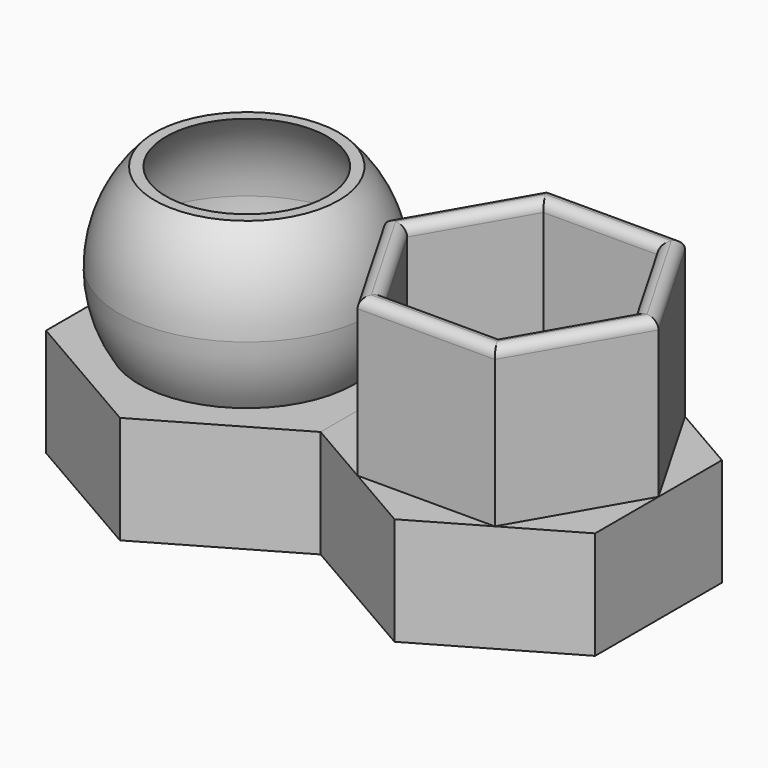
from build123d import *

# Parameters (mm, degrees)
F1_DEPTH        = 34.925
F3_DEPTH        = 50.8
F4_T            = 6.477
F4_T3_DEPTH     = 57.404
F4_T5_DEPTH     = 57.404
F4_T7_DEPTH     = 57.404
F4_T9_DEPTH     = 57.404
F4_T11_DEPTH    = 57.404
F5_R            = 3.23849
F6_R            = 9.5504
F7_DEPTH        = 5.334
F7_COPIES_COUNT = 6
F9_DEPTH        = 34.925
F15_T           = -2.54
F16_W           = 90.7614380121
F16_H           = 120.473433286
F17_DEPTH       = 25.4


# Not quite as in the source:
# - a fillet or chamfer is up to 0.001 mm smaller than in the source, because OpenCascade refuses the exact size
# - a pattern or mirror of a feature is missing from the dataset's text; its kind, count and spacing are read off the source's solid
# - a shell that OpenCascade refuses in one call is made with other operations: the cavity is built on its own and cut out


with BuildPart() as f1:
    # F0 (on Top) → F1 (new body)
    with BuildSketch(Plane.XY):
        Polygon((44.45, 25.6632194655), (0, 51.326438931), (-44.45, 25.6632194655), (-44.45, -25.6632194655), (0, -51.326438931), (44.45, -25.6632194655), align=None)
    extrude(amount=F1_DEPTH)

    # F2 (on face) → F3 (join)
    with BuildSketch(Plane.XY.offset(34.925)):
        Polygon((44.45, 0), (22.225, 38.4948291982), (-22.225, 38.4948291982), (-44.45, 0), (-22.225, -38.4948291982), (22.225, -38.4948291982), align=None)
    extrude(amount=F3_DEPTH)

    # F4: shell of thickness 6.477, made by hand


with BuildPart() as f4_core1:
    # F4_t2: copy of F1
    add(f1.part)

    # the walls: a layer under each face that stays
    f4_faces = [f4_core1.faces().sort_by_distance(p)[0] for p in [
        (22.225, 38.4948291982, 17.4625),
        (44.45, 0, 17.4625),
        (-22.225, 38.4948291982, 17.4625),
        (0, 0, 0),
        (40.7458333333, 19.2474145991, 34.925),
        (0, 44.9106340646, 34.925),
        (22.225, -38.4948291982, 17.4625),
        (40.7458333333, -19.2474145991, 34.925),
        (-44.45, 0, 17.4625),
        (-40.7458333333, 19.2474145991, 34.925),
        (-22.225, -38.4948291982, 17.4625),
        (33.3375, 19.2474145991, 60.325),
        (0, 38.4948291982, 60.325),
        (0, -44.9106340646, 34.925),
        (33.3375, -19.2474145991, 60.325),
        (-40.7458333333, -19.2474145991, 34.925),
        (-33.3375, 19.2474145991, 60.325),
        (0, -38.4948291982, 60.325),
        (-33.3375, -19.2474145991, 60.325),
    ]]
    thicken(f4_faces, amount=-F4_T, mode=Mode.SUBTRACT)

    # F4_s4 → F4_t3 (cut)
    with BuildSketch(Plane(origin=(14.351, -24.8566611394, 0), x_dir=(0, 0, 1), z_dir=(-0.5, 0.8660254038, 0))):
        Polygon((34.98977, 38.5595991982), (28.448, 38.4948291982), (28.448, 32.0178291982), (34.925, 32.0178291982), align=None)
    extrude(amount=F4_T3_DEPTH, mode=Mode.SUBTRACT)

    # F4_s6 → F4_t5 (cut)
    with BuildSketch(Plane.YZ.offset(-28.702)):
        Polygon((38.5595991982, 34.98977), (38.4948291982, 28.448), (32.0178291982, 28.448), (32.0178291982, 34.925), align=None)
        Polygon((-38.5595991982, 34.98977), (-38.4948291982, 28.448), (-32.0178291982, 28.448), (-32.0178291982, 34.925), align=None)
    extrude(amount=F4_T5_DEPTH, mode=Mode.SUBTRACT)

    # F4_s8 → F4_t7 (cut)
    with BuildSketch(Plane(origin=(-14.351, -24.8566611394, 0), x_dir=(0, 0, 1), z_dir=(0.5, 0.8660254038, 0))):
        Polygon((34.98977, 38.5595991982), (28.448, 38.4948291982), (28.448, 32.0178291982), (34.925, 32.0178291982), align=None)
    extrude(amount=F4_T7_DEPTH, mode=Mode.SUBTRACT)

    # F4_s10 → F4_t9 (cut)
    with BuildSketch(Plane(origin=(14.351, 24.8566611394, 0), x_dir=(0, 0, 1), z_dir=(-0.5, -0.8660254038, 0))):
        Polygon((34.98977, 38.5595991982), (28.448, 38.4948291982), (28.448, 32.0178291982), (34.925, 32.0178291982), align=None)
    extrude(amount=F4_T9_DEPTH, mode=Mode.SUBTRACT)

    # F4_s12 → F4_t11 (cut)
    with BuildSketch(Plane(origin=(-14.351, 24.8566611394, 0), x_dir=(0, 0, 1), z_dir=(0.5, -0.8660254038, 0))):
        Polygon((34.98977, 38.5595991982), (28.448, 38.4948291982), (28.448, 32.0178291982), (34.925, 32.0178291982), align=None)
    extrude(amount=F4_T11_DEPTH, mode=Mode.SUBTRACT)


with BuildPart() as f1_1:
    add(f1.part)

    # what is left inside the walls is the cavity
    f4_cavity = [f4_core1.part.solids().sort_by_distance(p)[0] for p in [
        (0, -14.615815, 6.54177),
    ]]
    add(f4_cavity, mode=Mode.SUBTRACT)

    # F5 (radius 3.2385 in the source; OpenCascade refuses exactly that, so slightly less here)
    f5_edges = [f1_1.edges().sort_by_distance(p)[0] for p in [
        (33.3375, -19.247415, 85.725),
        (0, -38.494829, 85.725),
        (33.3375, 19.247415, 85.725),
        (-33.3375, -19.247415, 85.725),
        (0, 38.494829, 85.725),
        (-33.3375, 19.247415, 85.725),
        (27.728253, -16.008915, 85.725),
        (27.728253, 16.008915, 85.725),
        (0, 32.017829, 85.725),
        (-27.728253, 16.008915, 85.725),
        (-27.728253, -16.008915, 85.725),
        (0, -32.017829, 85.725),
    ]]
    fillet(f5_edges, radius=F5_R)

    # F6 (on face) → F7 (cut)
    with BuildSketch(Plane(origin=(18.9865, -32.8855826579, 0), x_dir=(-0.8660254038, -0.5, 0), z_dir=(-0.5, 0.8660254038, 0))):
        with Locations((0, 17.4625)):
            Circle(F6_R)
    f7 = extrude(amount=-F7_DEPTH, mode=Mode.SUBTRACT)

    # F7_copies: F7 ×6 about axis
    f7_copies_axis = Axis((0, 0, 0), (0, 0, 1))
    for i in range(1, F7_COPIES_COUNT):
        add(f7.rotate(f7_copies_axis, i * 360 / F7_COPIES_COUNT), mode=Mode.SUBTRACT)


with BuildPart() as f9:
    # F8 (on Top) → F9 (new body)
    with BuildSketch(Plane.XY):
        Polygon((-44.45, -25.6632194655), (-44.45, 25.6632194655), (-88.9, 51.326438931), (-133.35, 25.6632194655), (-133.35, -25.6632194655), (-88.9, -51.326438931), align=None)
    extrude(amount=F9_DEPTH)

    # F10 (on Front) → F12 (revolve)
    with BuildSketch(Plane.XZ):
        with BuildLine():
            ThreePointArc((-88.9, 15.875), (-59.7141676065, 27.9641676065), (-47.625, 57.15))
            ThreePointArc((-47.625, 57.15), (-59.7141676065, 86.3358323935), (-88.9, 98.425))
            Line((-88.9, 98.425), (-88.9, 15.875))
        make_face()
    revolve(axis=Axis((-88.9, 0, 57.15), (0, 0, -1)))

    # F13 (on Front) → F14 (revolve, cut)
    with BuildSketch(Plane.XZ):
        with BuildLine():
            ThreePointArc((-88.9, 82.55), (-77.6746798487, 87.1996798487), (-73.025, 98.425))
            ThreePointArc((-73.025, 98.425), (-77.6746798487, 109.6503201513), (-88.9, 114.3))
            Line((-88.9, 114.3), (-88.9, 82.55))
        make_face()
    revolve(axis=Axis((-88.9, 0, 98.425), (0, 0, 1)), mode=Mode.SUBTRACT)

    # F15
    f15_openings = [f9.faces().sort_by_distance(p)[0] for p in [
        (-98.988386, 0, 86.167754),
    ]]
    offset(amount=F15_T, openings=f15_openings, kind=Kind.INTERSECTION)

    # F16 (on offset) → F17 (cut)
    with BuildSketch(Plane.XY.offset(85.725)):
        with Locations((-92.8241088986, -15.1389669627)):
            Rectangle(F16_W, F16_H)
    extrude(amount=F17_DEPTH, mode=Mode.SUBTRACT)


solid = Compound([f1_1.part, f9.part])
